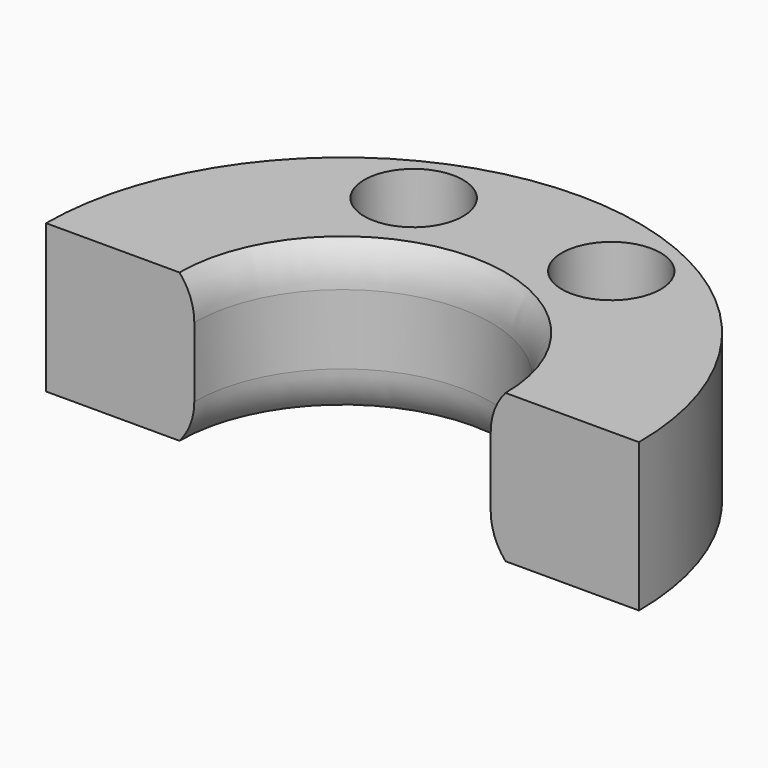
from build123d import *

# Parameters (mm, degrees)
F1_DEPTH    = 30
F2_R        = 6.5
F3_DEPTH    = 30
F4_R        = 10
F5_DEPTH    = 12
F6_R        = 10
F7_DEPTH    = 12
F8_SIZE     = 3
F9_T2_ANGLE = 227.2231239027
F9_T4_ANGLE = 227.2231239027


# Not quite as in the source:
# - a fillet or chamfer that OpenCascade refuses, or shapes differently, is made with other operations: its cross-section is extruded or revolved along the edge and cut away or added


with BuildPart() as f1:
    # F0 (on Top) → F1 (new body)
    with BuildSketch(Plane.XY):
        with BuildLine():
            Line((30, 0), (60, 0))
            ThreePointArc((60, 0), (0, 60), (-60, 0))
            Line((-60, 0), (-30, 0))
            ThreePointArc((-30, 0), (0, 30), (30, 0))
        make_face()
    extrude(amount=-F1_DEPTH)

    # F2 (on face) → F3 (cut, through all)
    with BuildSketch(Plane.XY):
        with Locations((20, 43)):
            Circle(F2_R)
        with Locations((-20, 43)):
            Circle(F2_R)
    extrude(amount=-F3_DEPTH, mode=Mode.SUBTRACT)

    # F4 (on face) → F5 (cut)
    with BuildSketch(Plane.XY):
        with Locations((20, 43)):
            Circle(F4_R)
        with Locations((-20, 43)):
            Circle(F4_R)
    extrude(amount=-F5_DEPTH, mode=Mode.SUBTRACT)

    # F6 (on face) → F7 (cut)
    with BuildSketch(Plane(origin=(0, 0, -30), x_dir=(1, 0, 0), z_dir=(0, 0, -1))):
        with Locations((-20, -43)):
            Circle(F6_R)
        with Locations((20, -43)):
            Circle(F6_R)
    extrude(amount=-F7_DEPTH, mode=Mode.SUBTRACT)

    # F8
    f8_edges = [f1.edges().sort_by_distance(p)[0] for p in [
        (0, 30, -30),
        (0, 30, 0),
    ]]
    chamfer(f8_edges, length=F8_SIZE)

    # F9: fillet of radius 12 on 2 edges, made by hand

    # F9_s1 → F9_t2 (revolve, cut)
    with BuildSketch(Plane(origin=(0, 0, 0), x_dir=(0, 0, 1), z_dir=(0.400533941, -0.9162819228, 0))):
        with BuildLine():
            ThreePointArc((-22.0627460668, 30), (-26.3053867539, 30.7750278397), (-30, 33))
            Line((-30, 33), (-27, 30))
            Line((-27, 30), (-22.0627460668, 30))
        make_face()
    revolve(axis=Axis((0, 0, -27), (0, 0, -1)), revolution_arc=F9_T2_ANGLE, mode=Mode.SUBTRACT)

    # F9_s3 → F9_t4 (revolve, cut)
    with BuildSketch(Plane(origin=(0, 0, 0), x_dir=(0, 0, 1), z_dir=(0.400533941, -0.9162819228, 0))):
        with BuildLine():
            ThreePointArc((-7.9372539332, 30), (-3.6946132461, 30.7750278397), (0, 33))
            Line((0, 33), (-3, 30))
            Line((-3, 30), (-7.9372539332, 30))
        make_face()
    revolve(axis=Axis((0, 0, -3), (0, 0, -1)), revolution_arc=F9_T4_ANGLE, mode=Mode.SUBTRACT)


solid = f1.part
